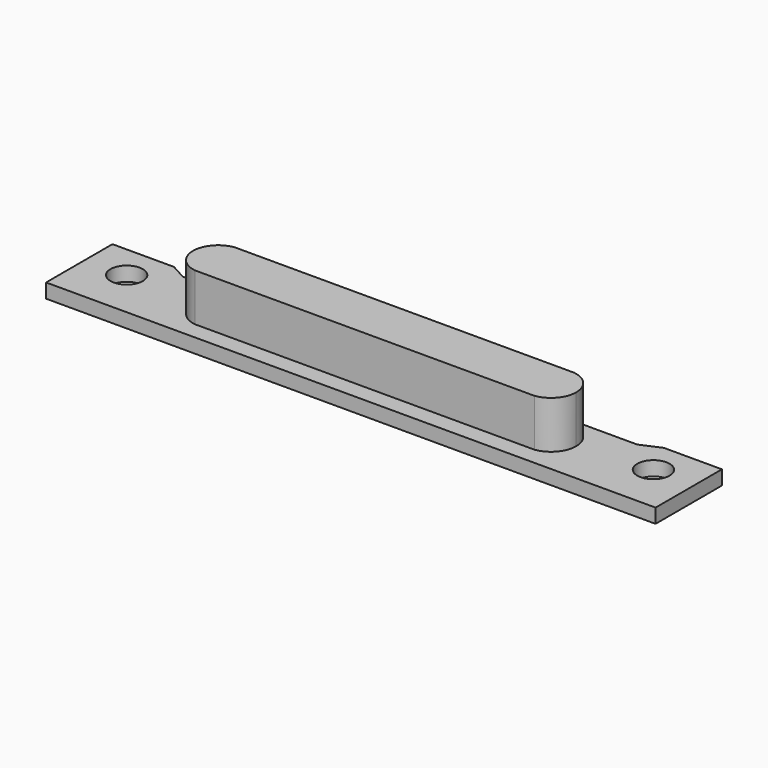
from build123d import *

# Parameters (mm, degrees)
F0_W     = 23
F0_H     = 3.13
F2_DEPTH = 0.54
F1_R     = 0.61
F3_DEPTH = 0.54
F5_DEPTH = 2.33
F7_DEPTH = 25


# Not quite as in the source:
# - a feature names something its author has since deleted; it is built from what else it names


with BuildPart() as f2:
    # F0 (on Top) → F2 (new body)
    with BuildSketch(Plane.XY):
        with Locations((-13.1842952464, 6.1040417799)):
            Rectangle(F0_W, F0_H)
    extrude(amount=F2_DEPTH)

    # F1 (on Top) → F3 (cut)
    with BuildSketch(Plane.XY):
        with Locations((-23.1242952464, 6.3890417799)):
            Circle(F1_R)
        with Locations((-3.2442952464, 6.3890417799)):
            Circle(F1_R)
    extrude(amount=F3_DEPTH, mode=Mode.SUBTRACT)

    # F6 (on Top) → F7 (cut)
    with BuildSketch(Plane.XY):
        Polygon((-3.7328053731, 8.1115094945), (-22.4673096091, 8.1115094945), (-22.4673096091, 7.7279869001), (-21.7720177025, 7.3444643058), (-4.6212589368, 7.3444643058), (-3.7328053731, 7.7279869001), align=None)
    extrude(amount=F7_DEPTH, mode=Mode.SUBTRACT)


with BuildPart() as f5:
    # F4 (on Top) → F5 (new body)
    with BuildSketch(Plane.XY):
        with BuildLine():
            ThreePointArc((-20.4164541145, 6.1365935627), (-20.1821228313, 5.5118830758), (-19.5947457105, 5.1953985412))
            Line((-19.5947457105, 5.1953985412), (-6.7784807016, 5.1953985412))
            ThreePointArc((-6.7784807016, 5.1953985412), (-6.1911035808, 5.5118830758), (-5.9567722976, 6.1365935627))
            ThreePointArc((-5.9567722976, 6.1365935627), (-6.1911035808, 6.7613040496), (-6.7784807016, 7.0777885842))
            Line((-6.7784807016, 7.0777885842), (-19.5947457105, 7.0777885842))
            ThreePointArc((-19.5947457105, 7.0777885842), (-20.1821228313, 6.7613040496), (-20.4164541145, 6.1365935627))
        make_face()
    extrude(amount=F5_DEPTH)


solid = Compound([f2.part, f5.part])
